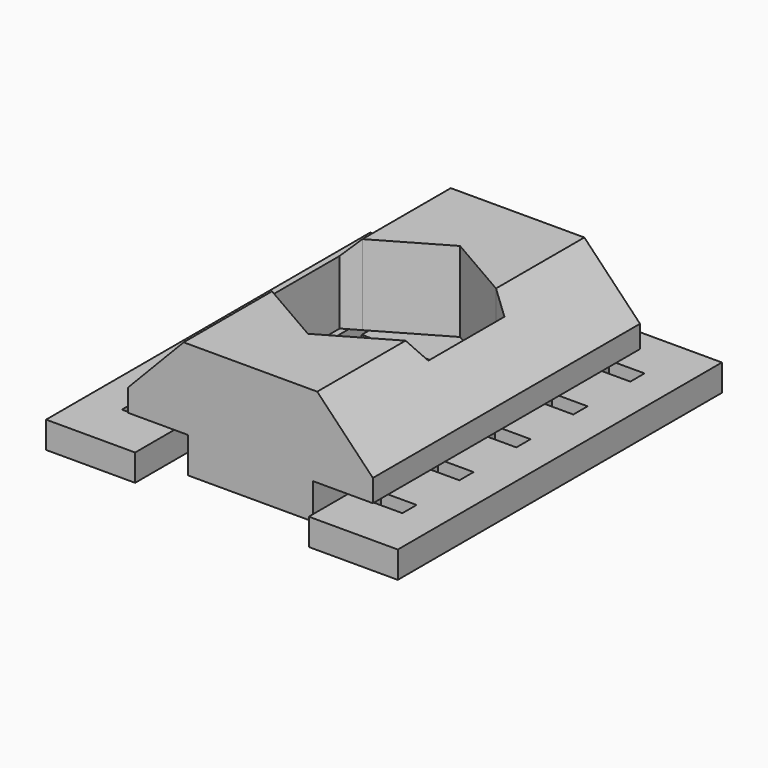
from build123d import *

# Parameters (mm, degrees)
F1_DEPTH = 15
F3_DEPTH = 3.6
F4_W     = 1.6
F4_H     = 0.8
F5_DEPTH = 1.2
F4_W_2   = 5.6
F4_H_2   = 4.5
F6_DEPTH = 1.6


# Not quite as in the source:
# - a feature names something its author has since deleted; it is built from what else it names


with BuildPart() as f1:
    # F0 (on Front) → F1 (new body)
    with BuildSketch(Plane.XZ):
        Polygon((-2.8, 0), (0, 0), (2.8, 0), (2.8, 1.6), (5.5, 1.6), (5.5, 2.6), (3, 5.2), (0, 5.2), (-3, 5.2), (-5.5, 2.6), (-5.5, 1.6), (-2.8, 1.6), align=None)
    extrude(amount=F1_DEPTH)

    # F2 (on face) → F3 (cut, through all)
    with BuildSketch(Plane.XY.offset(5.2)):
        Polygon((3, -4.9596588156), (0, -3.227608008), (-3, -4.9596588156), (-3, -10.0403411844), (0, -11.772391992), (3, -10.0403411844), align=None)
        Polygon((3.7, -5.363804004), (3, -4.9596588156), (3, -10.0403411844), (3.7, -9.636195996), align=None)
        Polygon((-3, -10.0403411844), (-3, -4.9596588156), (-3.7, -5.363804004), (-3.7, -9.636195996), align=None)
    extrude(amount=-F3_DEPTH, mode=Mode.SUBTRACT)

    # F4 (on Top) → F6 (cut, through all)
    with BuildSketch(Plane.XY):
        with Locations((0, -7.5)):
            Rectangle(F4_W_2, F4_H_2)
    extrude(amount=F6_DEPTH, mode=Mode.SUBTRACT)


with BuildPart() as f5:
    # F4 (on Top) → F5 (new body)
    with BuildSketch(Plane.XY):
        Polygon((-3.9, -0.743646355), (-3.9, 1.6), (-7.9, 1.6), (-7.9, -16.6), (-3.9, -16.6), (-3.9, -14.343646355), (-3.9, -13.543646355), (-3.9, -12.743646355), (-3.9, -11.943646355), (-3.9, -11.143646355), (-3.9, -10.343646355), (-3.9, -9.543646355), (-3.9, -8.743646355), (-3.9, -7.943646355), (-3.9, -7.143646355), (-3.9, -6.343646355), (-3.9, -5.543646355), (-3.9, -4.743646355), (-3.9, -3.943646355), (-3.9, -3.143646355), (-3.9, -2.343646355), (-3.9, -1.543646355), align=None)
        with Locations((-5.5, -13.943646355)):
            Rectangle(F4_W, F4_H, mode=Mode.SUBTRACT)
        with Locations((-5.5, -10.743646355)):
            Rectangle(F4_W, F4_H, mode=Mode.SUBTRACT)
        with Locations((-5.5, -7.543646355)):
            Rectangle(F4_W, F4_H, mode=Mode.SUBTRACT)
        with Locations((-5.5, -4.343646355)):
            Rectangle(F4_W, F4_H, mode=Mode.SUBTRACT)
        with Locations((-5.5, -1.143646355)):
            Rectangle(F4_W, F4_H, mode=Mode.SUBTRACT)
    extrude(amount=F5_DEPTH)


with BuildPart() as f7_1:
    # F7: instance of F5
    add(f5.part.mirror(Plane.YZ))


solid = Compound([f1.part, f5.part, f7_1.part])
